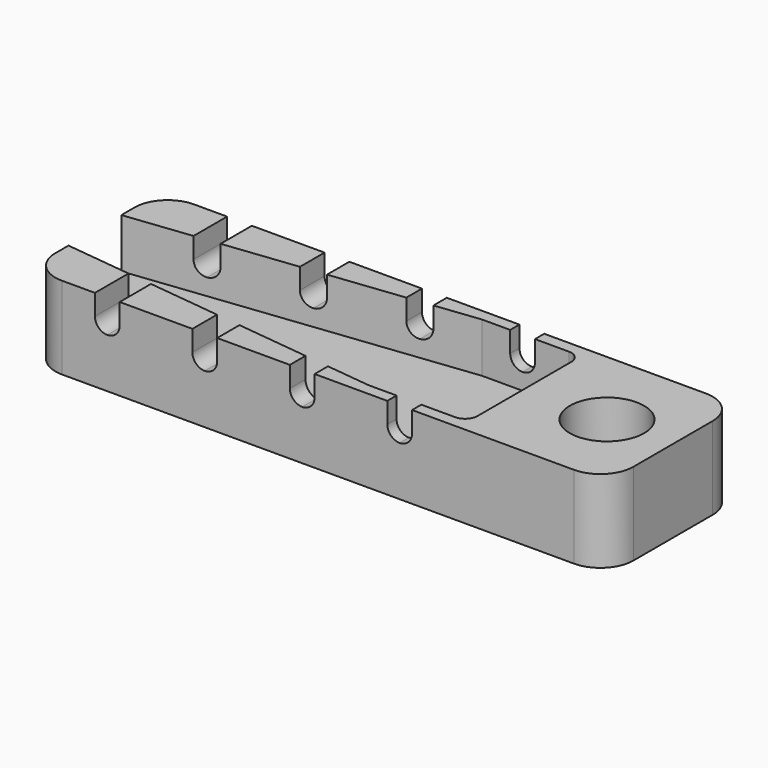
from build123d import *

# Parameters (mm, degrees)
F0_W     = 1.5
F0_H     = 0.7
F0_R     = 2.25
F0_H_2   = 8.6
F0_W_2   = 2.8
F1_DEPTH = 5
F2_DEPTH = 3
F3_DEPTH = 2
F4_R     = 0.74999
F5_R     = 2


# Not quite as in the source:
# - a fillet or chamfer is up to 0.001 mm smaller than in the source, because OpenCascade refuses the exact size


with BuildPart() as f1:
    # F0 (on Top) → F1 (new body)
    with BuildSketch(Plane.XY):
        Polygon((-18.8879279066, 5), (-22.8879279066, 5), (-22.8879279066, 2), (-18.8879279066, 2.46), align=None)
        Polygon((-17.3879279066, 5), (-18.8879279066, 5), (-18.8879279066, 2.46), (-17.3879279066, 2.6325), align=None)
        Polygon((-18.8879279066, 2.46), (-22.8879279066, 2), (-22.8879279066, -2), (-18.8879279066, -2.46), align=None)
        Polygon((-12.9879279066, 5), (-17.3879279066, 5), (-17.3879279066, 2.6325), (-12.9879279066, 3.1385), align=None)
        Polygon((-18.8879279066, -2.46), (-22.8879279066, -2), (-22.8879279066, -5), (-18.8879279066, -5), align=None)
        Polygon((-11.4879279066, 5), (-12.9879279066, 5), (-12.9879279066, 3.1385), (-11.4879279066, 3.311), align=None)
        Polygon((-17.3879279066, -2.6325), (-18.8879279066, -2.46), (-18.8879279066, -5), (-17.3879279066, -5), align=None)
        Polygon((-7.0879279066, 5), (-11.4879279066, 5), (-11.4879279066, 3.311), (-7.0879279066, 3.817), align=None)
        Polygon((-12.9879279066, -3.1385), (-17.3879279066, -2.6325), (-17.3879279066, -5), (-12.9879279066, -5), align=None)
        Polygon((-5.5879279066, 5), (-7.0879279066, 5), (-7.0879279066, 3.817), (-5.5879279066, 3.9895), align=None)
        Polygon((-11.4879279066, -3.311), (-12.9879279066, -3.1385), (-12.9879279066, -5), (-11.4879279066, -5), align=None)
        Polygon((-1.1879279066, 5), (-5.5879279066, 5), (-5.5879279066, 3.9895), (-2.8879279066, 4.3), (-1.1879279066, 4.3), align=None)
        Polygon((-7.0879279066, -3.817), (-11.4879279066, -3.311), (-11.4879279066, -5), (-7.0879279066, -5), align=None)
        with Locations((-0.4379279066, 4.65)):
            Rectangle(F0_W, F0_H)
        Polygon((-5.5879279066, -3.9895), (-7.0879279066, -3.817), (-7.0879279066, -5), (-5.5879279066, -5), align=None)
        Polygon((12.1120720934, 5), (0.3120720934, 5), (0.3120720934, 4.3), (3.1120720934, 4.3), (3.1120720934, -4.3), (0.3120720934, -4.3), (0.3120720934, -5), (12.1120720934, -5), align=None)
        with Locations((8.1120720934, 0)):
            Circle(F0_R, mode=Mode.SUBTRACT)
        Polygon((-2.8879279066, -4.3), (-5.5879279066, -3.9895), (-5.5879279066, -5), (-1.1879279066, -5), (-1.1879279066, -4.3), align=None)
        with Locations((-0.4379279066, -4.65)):
            Rectangle(F0_W, F0_H)
        with Locations((-0.4379279066, 0)):
            Rectangle(F0_W, F0_H_2)
        Polygon((-5.5879279066, 3.9895), (-7.0879279066, 3.817), (-7.0879279066, -3.817), (-5.5879279066, -3.9895), align=None)
        Polygon((-17.3879279066, 2.6325), (-18.8879279066, 2.46), (-18.8879279066, -2.46), (-17.3879279066, -2.6325), align=None)
        Polygon((-12.9879279066, 3.1385), (-17.3879279066, 2.6325), (-17.3879279066, -2.6325), (-12.9879279066, -3.1385), align=None)
        Polygon((-7.0879279066, 3.817), (-11.4879279066, 3.311), (-11.4879279066, -3.311), (-7.0879279066, -3.817), align=None)
        Polygon((-11.4879279066, 3.311), (-12.9879279066, 3.1385), (-12.9879279066, -3.1385), (-11.4879279066, -3.311), align=None)
        Polygon((-2.8879279066, 4.3), (-5.5879279066, 3.9895), (-5.5879279066, -3.9895), (-2.8879279066, -4.3), (-1.1879279066, -4.3), (-1.1879279066, 4.3), align=None)
        with Locations((1.7120720934, 0)):
            Rectangle(F0_W_2, F0_H_2)
    extrude(amount=-F1_DEPTH)

    # F0 (on Top) → F2 (cut)
    with BuildSketch(Plane.XY):
        Polygon((-18.8879279066, 2.46), (-22.8879279066, 2), (-22.8879279066, -2), (-18.8879279066, -2.46), align=None)
        Polygon((-17.3879279066, 2.6325), (-18.8879279066, 2.46), (-18.8879279066, -2.46), (-17.3879279066, -2.6325), align=None)
        Polygon((-12.9879279066, 3.1385), (-17.3879279066, 2.6325), (-17.3879279066, -2.6325), (-12.9879279066, -3.1385), align=None)
        Polygon((-11.4879279066, 3.311), (-12.9879279066, 3.1385), (-12.9879279066, -3.1385), (-11.4879279066, -3.311), align=None)
        Polygon((-7.0879279066, 3.817), (-11.4879279066, 3.311), (-11.4879279066, -3.311), (-7.0879279066, -3.817), align=None)
        Polygon((-5.5879279066, 3.9895), (-7.0879279066, 3.817), (-7.0879279066, -3.817), (-5.5879279066, -3.9895), align=None)
        Polygon((-2.8879279066, 4.3), (-5.5879279066, 3.9895), (-5.5879279066, -3.9895), (-2.8879279066, -4.3), (-1.1879279066, -4.3), (-1.1879279066, 4.3), align=None)
        with Locations((-0.4379279066, 0)):
            Rectangle(F0_W, F0_H_2)
        with Locations((1.7120720934, 0)):
            Rectangle(F0_W_2, F0_H_2)
    extrude(amount=-F2_DEPTH, mode=Mode.SUBTRACT)

    # F0 (on Top) → F3 (cut)
    with BuildSketch(Plane.XY):
        Polygon((-17.3879279066, 5), (-18.8879279066, 5), (-18.8879279066, 2.46), (-17.3879279066, 2.6325), align=None)
        Polygon((-11.4879279066, 5), (-12.9879279066, 5), (-12.9879279066, 3.1385), (-11.4879279066, 3.311), align=None)
        Polygon((-5.5879279066, 5), (-7.0879279066, 5), (-7.0879279066, 3.817), (-5.5879279066, 3.9895), align=None)
        with Locations((-0.4379279066, -4.65)):
            Rectangle(F0_W, F0_H)
        Polygon((-17.3879279066, -2.6325), (-18.8879279066, -2.46), (-18.8879279066, -5), (-17.3879279066, -5), align=None)
        Polygon((-11.4879279066, -3.311), (-12.9879279066, -3.1385), (-12.9879279066, -5), (-11.4879279066, -5), align=None)
        Polygon((-5.5879279066, -3.9895), (-7.0879279066, -3.817), (-7.0879279066, -5), (-5.5879279066, -5), align=None)
        with Locations((-0.4379279066, 4.65)):
            Rectangle(F0_W, F0_H)
    extrude(amount=-F3_DEPTH, mode=Mode.SUBTRACT)

    # F4 (radius 0.75 in the source; OpenCascade refuses exactly that, so slightly less here)
    f4_edges = [f1.edges().sort_by_distance(p)[0] for p in [
        (-17.387928, -3.81625, -2),
        (-11.487928, -4.1555, -2),
        (-5.587928, -4.49475, -2),
        (0.312072, -4.65, -2),
        (-18.887928, -3.73, -2),
        (-12.987928, -4.06925, -2),
        (-7.087928, -4.4085, -2),
        (-1.187928, -4.65, -2),
        (-18.887928, 3.73, -2),
        (-12.987928, 4.06925, -2),
        (-7.087928, 4.4085, -2),
        (-1.187928, 4.65, -2),
        (-17.387928, 3.81625, -2),
        (-11.487928, 4.1555, -2),
        (-5.587928, 4.49475, -2),
        (0.312072, 4.65, -2),
        (3.112072, 4.3, -1.5),
        (3.112072, -4.3, -1.5),
    ]]
    fillet(f4_edges, radius=F4_R)

    # F5
    f5_edges = [f1.edges().sort_by_distance(p)[0] for p in [
        (-22.887928, -5, -2.5),
        (-22.887928, 5, -2.5),
        (12.112072, -5, -2.5),
        (12.112072, 5, -2.5),
    ]]
    fillet(f5_edges, radius=F5_R)


solid = f1.part
